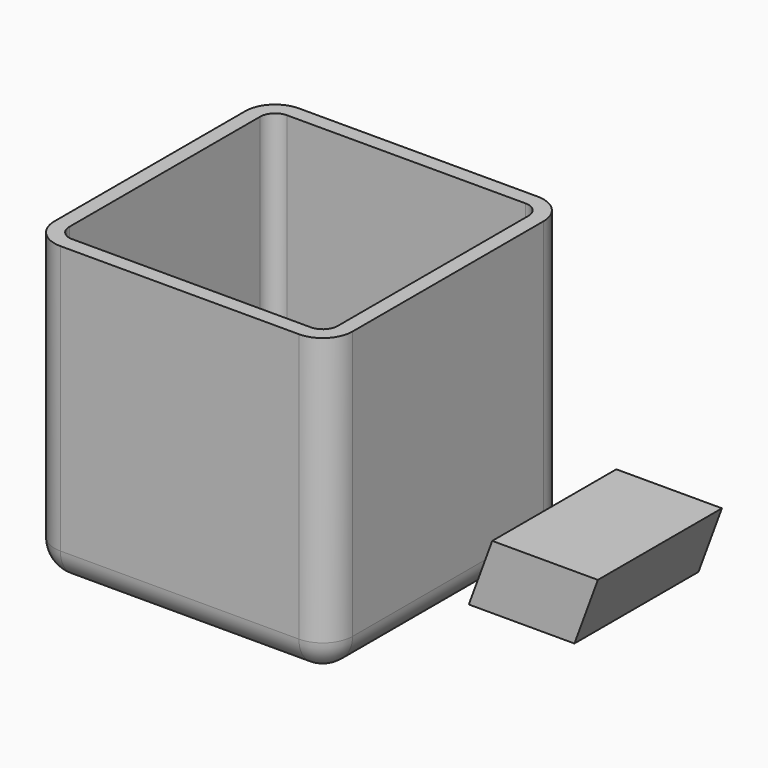
from build123d import *

# Parameters (mm, degrees)
F1_DEPTH        = 52
F2_W            = 100
F2_H            = 100
F3_DEPTH        = 100
F4_R            = 10
F5_T            = -5
F6_R            = 3
F7_DEPTH        = 25
F8_R            = 3
F9_DEPTH        = 25
F9_COPIES_COUNT = 4


# Not quite as in the source:
# - a pattern or mirror of a feature is missing from the dataset's text; its kind, count and spacing are read off the source's solid


with BuildPart() as f1:
    # F0 (on Front) → F1 (new body)
    with BuildSketch(Plane.XZ):
        Polygon((16.4231043309, 28.0736852437), (8.5624745116, 6.7376843654), (43.9754001059, 6.7376843654), (51.8360299253, 28.0736852437), align=None)
    extrude(amount=F1_DEPTH)


with BuildPart() as f3:
    # F2 (on Front) → F3 (new body)
    with BuildSketch(Plane.XZ):
        with Locations((-50, 50)):
            Rectangle(F2_W, F2_H)
    extrude(amount=F3_DEPTH)

    # F4
    f4_edges = [f3.edges().sort_by_distance(p)[0] for p in [
        (-100, 0, 50),
        (-100, -100, 50),
        (0, 0, 50),
        (0, -100, 50),
        (-50, -100, 0),
        (-100, -50, 0),
        (-50, 0, 0),
        (0, -50, 0),
    ]]
    fillet(f4_edges, radius=F4_R)

    # F5
    f5_openings = [f3.faces().sort_by_distance(p)[0] for p in [
        (-50, -50, 100),
    ]]
    offset(amount=F5_T, openings=f5_openings)

    # F6 (on face) → F7 (cut)
    with BuildSketch(Plane(origin=(0, 0, 0), x_dir=(1, 0, 0), z_dir=(0, 0, -1))):
        with Locations((-50, 50)):
            Circle(F6_R)
    extrude(amount=-F7_DEPTH, mode=Mode.SUBTRACT)

    # F8 (on face) → F9 (cut)
    with BuildSketch(Plane(origin=(0, 0, 0), x_dir=(1, 0, 0), z_dir=(0, 0, -1))):
        with Locations((-49.5, 22)):
            Circle(F8_R)
    f9 = extrude(amount=-F9_DEPTH, mode=Mode.SUBTRACT)

    # F9_copies: F9 ×4 about axis
    f9_copies_axis = Axis((-50, -50, 0), (0, 0, 1))
    for i in range(1, F9_COPIES_COUNT):
        add(f9.rotate(f9_copies_axis, i * 360 / F9_COPIES_COUNT), mode=Mode.SUBTRACT)


solid = Compound([f1.part, f3.part])
